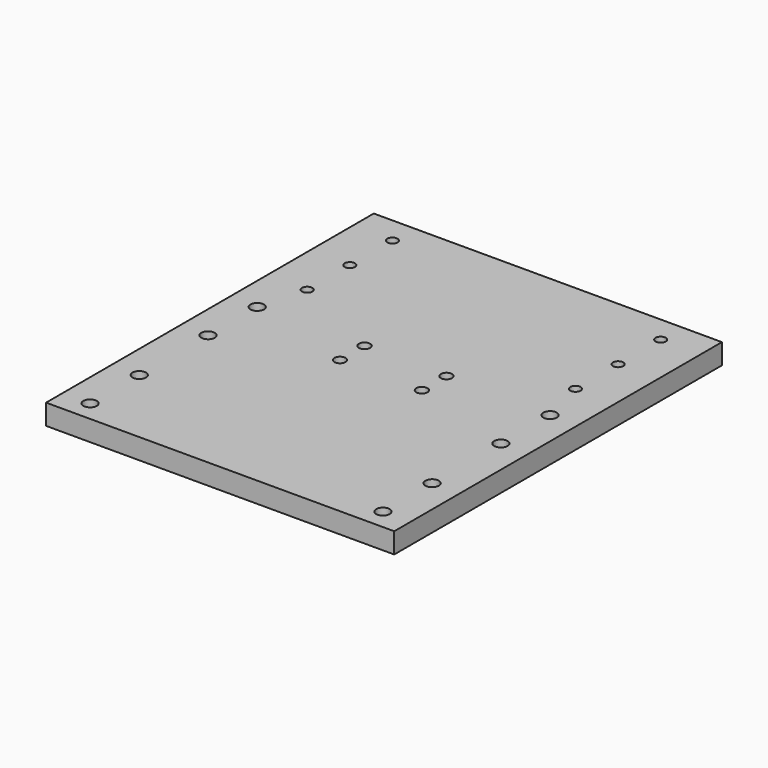
from build123d import *

# Parameters (mm, degrees)
F0_W           = 150
F0_H           = 200
F1_DEPTH       = 10
F3_D           = 5
F5_DEPTH       = 10
F6_DEPTH       = 10
F7_D           = 6.6
F7_CBORE_D     = 11.25
F7_CBORE_DEPTH = 6
F8_D           = 5.5
F8_CBORE_D     = 9.75
F8_CBORE_DEPTH = 5


# Not quite as in the source:
# - a feature names something its author has since deleted; it is built from what else it names


with BuildPart() as f1:
    # F0 (on Top) → F1 (new body)
    with BuildSketch(Plane.XY):
        with Locations((34.3934863061, 53.7353821645)):
            Rectangle(F0_W, F0_H)
    extrude(amount=F1_DEPTH)

    # F3 (through all)
    with Locations(Plane(origin=(0, 0, 0), x_dir=(1, 0, 0), z_dir=(0, 0, -1))):
        with Locations((-31.1065136939, -140.7353821645), (-31.1065136939, -114.7353821645), (-31.1065136939, -88.7353821645), (99.8934863061, -88.7353821645), (99.8934863061, -114.7353821645), (99.8934863061, -140.7353821645)):
            Hole(F3_D / 2)

    # F5 (add): a face of the model
    f5_faces = [f1.faces().sort_by_distance(p)[0] for p in [
        (109.3934863061, 53.7353821645, 5),
    ]]
    extrude(f5_faces, amount=F5_DEPTH)

    # F6 (add): a face of the model
    f6_faces = [f1.faces().sort_by_distance(p)[0] for p in [
        (-40.6065136939, 53.7353821645, 5),
    ]]
    extrude(f6_faces, amount=F6_DEPTH)

    # F7 (through all)
    with Locations(Plane(origin=(0, 0, 0), x_dir=(1, 0, 0), z_dir=(0, 0, -1))):
        with Locations((-37.1065136939, 36.2646178355), (-37.1065136939, 6.2646178355), (105.8934863061, 36.2646178355), (105.8934863061, 6.2646178355), (105.8934863061, -35.7353821645), (105.8934863061, -65.7353821645), (-37.1065136939, -65.7353821645), (-37.1065136939, -35.7353821645)):
            CounterBoreHole(F7_D / 2, F7_CBORE_D / 2, F7_CBORE_DEPTH)

    # F8 (through all)
    with Locations(Plane(origin=(0, 0, 0), x_dir=(1, 0, 0), z_dir=(0, 0, -1))):
        with Locations((54.8934863061, -51.2353821645), (54.8934863061, -66.2353821645), (14.8934863061, -51.2353821645), (14.8934863061, -66.2353821645)):
            CounterBoreHole(F8_D / 2, F8_CBORE_D / 2, F8_CBORE_DEPTH)


solid = f1.part
